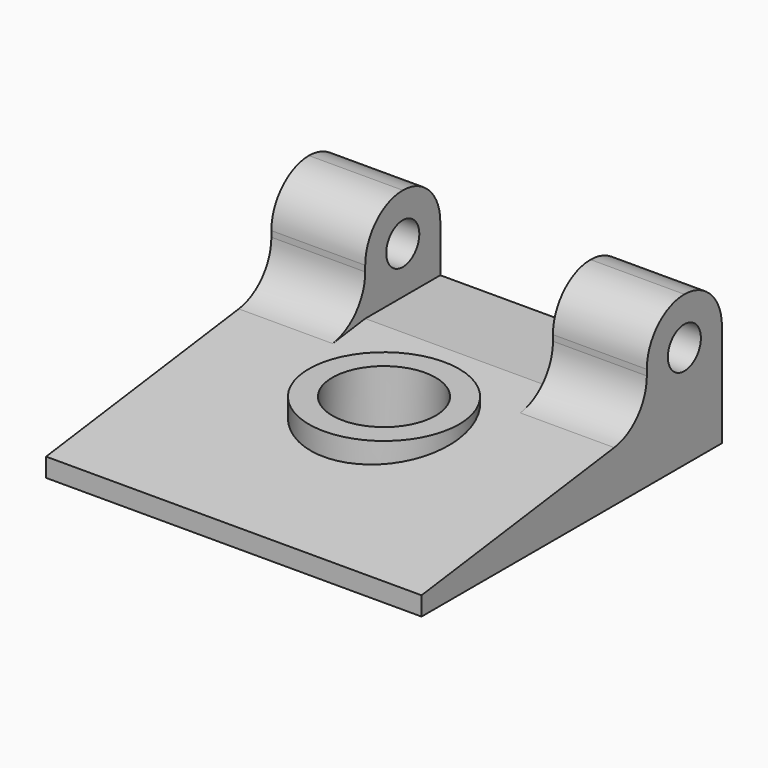
from build123d import *

# Parameters (mm, degrees)
F0_W        = 20
F0_H        = 20
F0_R        = 4
F1_DEPTH    = 4
F1_FACE_W   = 20
F1_FACE_H   = 20
F1_FACE_R   = 4
F0_R_2      = 2.75
F2_DEPTH    = 1
F3_W        = 5
F3_H        = 5
F4_DEPTH    = 5
F5_T1_DEPTH = 97.9746917615
F6_R        = 2.49999
F7_R        = 1.1
F8_DEPTH    = 25
F9_DEPTH    = 5
F10_DEPTH   = 2
F11_DEPTH   = 2


# Not quite as in the source:
# - a fillet or chamfer that OpenCascade refuses, or shapes differently, is made with other operations: its cross-section is extruded or revolved along the edge and cut away or added
# - a fillet or chamfer is up to 0.001 mm smaller than in the source, because OpenCascade refuses the exact size


with BuildPart() as f1:
    # F0 (on Top) → F1 (new body)
    with BuildSketch(Plane.XY):
        with Locations((10, 10)):
            Rectangle(F0_W, F0_H)
        with Locations((10, 10)):
            Circle(F0_R, mode=Mode.SUBTRACT)
    extrude(amount=F1_DEPTH)

    # F1_face (on face) + F0 (on Top) → F2 (join)
    with BuildSketch(Plane(origin=(10, 10, 4), x_dir=(1, 0, 0), z_dir=(0, 0, 1))):
        Rectangle(F1_FACE_W, F1_FACE_H)
        Circle(F1_FACE_R, mode=Mode.SUBTRACT)
    with BuildSketch(Plane.XY):
        with Locations((10, 10)):
            Circle(F0_R)
        with Locations((10, 10)):
            Circle(F0_R_2, mode=Mode.SUBTRACT)
    extrude(amount=F2_DEPTH)

    # F3 (on face) → F4 (join)
    with BuildSketch(Plane.XY.offset(5)):
        with Locations((2.5, 17.5)):
            Rectangle(F3_W, F3_H)
        with Locations((17.5, 17.5)):
            Rectangle(F3_W, F3_H)
    extrude(amount=F4_DEPTH)

    # F5: chamfer of 15 x 2 on 1 edges, made by hand

    # F5_s2 → F5_t1 (cut)
    with BuildSketch(Plane.YZ.offset(-38.9873458808)):
        Polygon((0, 3), (15, 5), (0, 5), align=None)
    extrude(amount=F5_T1_DEPTH, mode=Mode.SUBTRACT)

    # F6 (radius 2.5 in the source; OpenCascade refuses exactly that, so slightly less here)
    f6_edges = [f1.edges().sort_by_distance(p)[0] for p in [
        (2.5, 15, 5),
        (2.5, 15, 10),
        (17.5, 15, 5),
        (17.5, 15, 10),
        (2.5, 20, 10),
        (17.5, 20, 10),
    ]]
    fillet(f6_edges, radius=F6_R)

    # F7 (on face) → F8 (cut)
    with BuildSketch(Plane(origin=(0, 0, 0), x_dir=(0, -1, 0), z_dir=(-1, 0, 0))):
        with Locations((-17.5, 7.5)):
            Circle(F7_R)
    extrude(amount=-F8_DEPTH, mode=Mode.SUBTRACT)

    # F0 (on Top) → F9 (join)
    with BuildSketch(Plane.XY):
        with Locations((10, 10)):
            Circle(F0_R)
        with Locations((10, 10)):
            Circle(F0_R_2, mode=Mode.SUBTRACT)
    extrude(amount=F9_DEPTH)

    # F0 (on Top) → F10 (join)
    with BuildSketch(Plane.XY):
        with Locations((10, 10)):
            Circle(F0_R_2)
    extrude(amount=F10_DEPTH)

    # F0 (on Top) → F11 (cut)
    with BuildSketch(Plane.XY):
        with Locations((10, 10)):
            Rectangle(F0_W, F0_H)
        with Locations((10, 10)):
            Circle(F0_R, mode=Mode.SUBTRACT)
        with Locations((10, 10)):
            Circle(F0_R)
        with Locations((10, 10)):
            Circle(F0_R_2, mode=Mode.SUBTRACT)
        with Locations((10, 10)):
            Circle(F0_R_2)
    extrude(amount=F11_DEPTH, mode=Mode.SUBTRACT)


solid = f1.part
